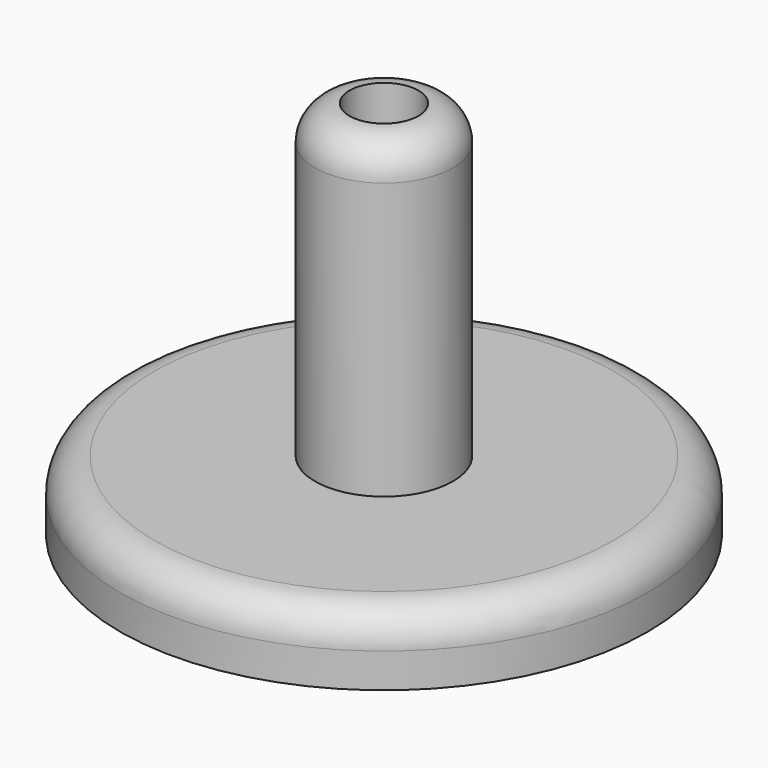
from build123d import *

# Parameters (mm, degrees)
F0_R     = 7.6516982388
F0_R_2   = 1
F2_DEPTH = 2
F1_R     = 2
F1_R_2   = 1
F3_DEPTH = 9
F4_R     = 0.99999
F5_R     = 1


# Not quite as in the source:
# - a fillet or chamfer is up to 0.001 mm smaller than in the source, because OpenCascade refuses the exact size


with BuildPart() as f2:
    # F0 (on Top) → F2 (new body)
    with BuildSketch(Plane.XY):
        Circle(F0_R)
        Circle(F0_R_2, mode=Mode.SUBTRACT)
    extrude(amount=-F2_DEPTH)

    # F1 (on face) → F3 (join)
    with BuildSketch(Plane.XY):
        Circle(F1_R)
        Circle(F1_R_2, mode=Mode.SUBTRACT)
    extrude(amount=F3_DEPTH)

    # F4 (radius 1 in the source; OpenCascade refuses exactly that, so slightly less here)
    f4_edges = [f2.edges().sort_by_distance(p)[0] for p in [
        (-2, 0, 9),
    ]]
    fillet(f4_edges, radius=F4_R)

    # F5
    f5_edges = [f2.edges().sort_by_distance(p)[0] for p in [
        (-7.651698, 0, 0),
    ]]
    fillet(f5_edges, radius=F5_R)


solid = f2.part
